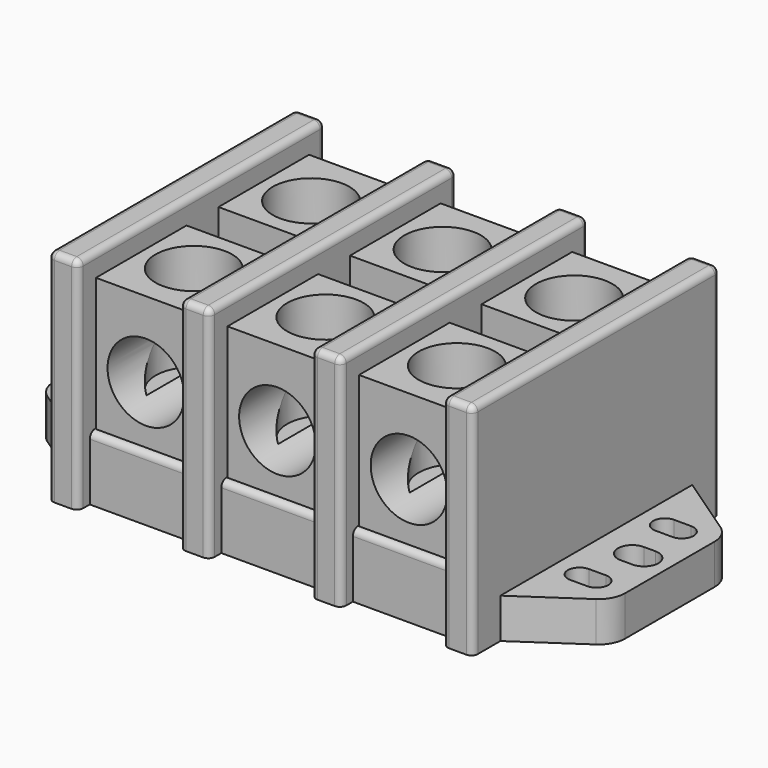
from build123d import *

# Parameters (mm, degrees)
F1_DEPTH  = 52.324
F0_W      = 7.14375
F0_H      = 73.66
F3_DEPTH  = 15.24
F5_DEPTH  = 9.525
F6_R      = 1.524
F6_2_R    = 1.524
F6_3_R    = 1.524
F6_4_R    = 1.524
F6_5_R    = 1.524
F8_DEPTH  = 9.525
F9_W      = 4.064
F9_H      = 5.588
F9_W_2    = 2.794
F9_H_2    = 6.858
F10_DEPTH = 9.525
F11_W     = 2.794
F11_H     = 6.858
F11_W_2   = 4.064
F11_H_2   = 5.588
F12_DEPTH = 9.525
F13_R     = 6.35
F13_2_R   = 6.35
F15_W     = 23.8125
F15_H     = 63.5
F18_DEPTH = 31.75
F16_W     = 23.8125
F16_H     = 63.5
F17_W     = 23.8125
F17_H     = 63.5
F19_R     = 9.128125
F20_DEPTH = 25.4
F21_R     = 9.128125
F22_DEPTH = 25.4
F23_R     = 9.128125
F24_DEPTH = 25.4
F25_W     = 23.8125
F25_H     = 9.525
F26_DEPTH = 18.034
F27_W     = 23.8125
F27_H     = 9.525
F28_DEPTH = 18.034
F29_W     = 23.8125
F29_H     = 9.525
F30_DEPTH = 18.034
F31_R     = 9.144
F32_DEPTH = 26.9875
F33_R     = 9.128125
F34_DEPTH = 26.9875
F35_R     = 9.128125
F36_DEPTH = 26.9875
F37_R     = 9.128125
F38_DEPTH = 26.9875
F39_R     = 9.128125
F40_DEPTH = 26.9875
F41_R     = 9.128125
F42_DEPTH = 26.9875


# Not quite as in the source:
# - a feature names something its author has since deleted; it is built from what else it names


with BuildPart() as f1:
    # F0 (on Top) → F1 (new body)
    with BuildSketch(Plane.XY):
        Polygon((-50.6015625, -36.83), (-43.4578125, -36.83), (-43.4578125, 36.83), (-50.6015625, 36.83), align=None)
    extrude(amount=F1_DEPTH)

    # F4 (on Top) → F5 (join)
    with BuildSketch(Plane.XY):
        Polygon((-50.6015625, -28.575), (-50.6015625, 28.575), (-68.1275625, 16.66875), (-68.1275625, -16.66875), align=None)
    extrude(amount=F5_DEPTH)

    # F6
    f6_edges = [f1.edges().sort_by_distance(p)[0] for p in [
        (-50.601563, 36.83, 26.162),
        (-50.601563, 0, 52.324),
        (-50.601563, -36.83, 26.162),
        (-43.457813, -36.83, 26.162),
        (-43.457813, 0, 52.324),
        (-47.029688, -36.83, 52.324),
        (-47.029687, 36.83, 52.324),
        (-43.457813, 36.83, 26.162),
    ]]
    fillet(f6_edges, radius=F6_R)

    # F9 (on face) → F10 (cut)
    with BuildSketch(Plane.XY.offset(9.525)):
        with Locations((-58.801, 12.7)):
            Rectangle(F9_W, F9_H)
        with BuildLine():
            Line((-56.769, 15.494), (-56.769, 9.906))
            ThreePointArc((-56.769, 9.906), (-53.975, 12.7), (-56.769, 15.494))
        make_face()
        with BuildLine():
            ThreePointArc((-60.833, 15.494), (-63.627, 12.7), (-60.833, 9.906))
            Line((-60.833, 9.906), (-60.833, 15.494))
        make_face()
        with Locations((-60.579, 0)):
            Rectangle(F9_W_2, F9_H_2)
        with BuildLine():
            Line((-59.182, 3.429), (-59.182, -3.429))
            ThreePointArc((-59.182, -3.429), (-55.753, 0), (-59.182, 3.429))
        make_face()
        with BuildLine():
            ThreePointArc((-61.976, 3.429), (-65.405, 0), (-61.976, -3.429))
            Line((-61.976, -3.429), (-61.976, 3.429))
        make_face()
        with Locations((-58.801, -12.7)):
            Rectangle(F9_W, F9_H)
        with BuildLine():
            Line((-56.769, -9.906), (-56.769, -15.494))
            ThreePointArc((-56.769, -15.494), (-53.975, -12.7), (-56.769, -9.906))
        make_face()
        with BuildLine():
            ThreePointArc((-60.833, -9.906), (-63.627, -12.7), (-60.833, -15.494))
            Line((-60.833, -15.494), (-60.833, -9.906))
        make_face()
    extrude(amount=-F10_DEPTH, mode=Mode.SUBTRACT)

    # F13
    f13_edges = [f1.edges().sort_by_distance(p)[0] for p in [
        (-68.127563, 16.66875, 4.7625),
        (-68.127563, -16.66875, 4.7625),
    ]]
    fillet(f13_edges, radius=F13_R)


with BuildPart() as f1b:
    # F0 (on Top) → F1, piece 2 (new body)
    with BuildSketch(Plane.XY):
        Polygon((43.4578125, 36.83), (43.4578125, -36.83), (50.6015625, -36.83), (50.6015625, 36.83), align=None)
    extrude(amount=F1_DEPTH)

    # F6#3
    f6_3_edges = [f1b.edges().sort_by_distance(p)[0] for p in [
        (43.457812, -36.83, 26.162),
        (50.601562, -36.83, 26.162),
        (47.029687, -36.83, 52.324),
        (43.457812, 0, 52.324),
        (50.601562, 0, 52.324),
        (47.029688, 36.83, 52.324),
        (43.457813, 36.83, 26.162),
        (50.601563, 36.83, 26.162),
    ]]
    fillet(f6_3_edges, radius=F6_3_R)

    # F7 (on Top) → F8 (join)
    with BuildSketch(Plane.XY):
        Polygon((68.1275625, 16.66875), (50.6015625, 28.575), (50.6015625, -28.575), (68.1275625, -16.66875), align=None)
    extrude(amount=F8_DEPTH)

    # F11 (on face) → F12 (cut)
    with BuildSketch(Plane.XY.offset(9.525)):
        with Locations((60.579, 0)):
            Rectangle(F11_W, F11_H)
        with BuildLine():
            ThreePointArc((59.182, 3.429), (55.753, 0), (59.182, -3.429))
            Line((59.182, -3.429), (59.182, 3.429))
        make_face()
        with BuildLine():
            Line((61.976, 3.429), (61.976, -3.429))
            ThreePointArc((61.976, -3.429), (65.405, 0), (61.976, 3.429))
        make_face()
        with Locations((58.801, 12.7)):
            Rectangle(F11_W_2, F11_H_2)
        with BuildLine():
            Line((60.833, 15.494), (60.833, 9.906))
            ThreePointArc((60.833, 9.906), (63.627, 12.7), (60.833, 15.494))
        make_face()
        with BuildLine():
            ThreePointArc((56.769, 15.494), (53.975, 12.7), (56.769, 9.906))
            Line((56.769, 9.906), (56.769, 15.494))
        make_face()
        with Locations((58.801, -12.7)):
            Rectangle(F11_W_2, F11_H_2)
        with BuildLine():
            Line((60.833, -9.906), (60.833, -15.494))
            ThreePointArc((60.833, -15.494), (63.627, -12.7), (60.833, -9.906))
        make_face()
        with BuildLine():
            ThreePointArc((56.769, -9.906), (53.975, -12.7), (56.769, -15.494))
            Line((56.769, -15.494), (56.769, -9.906))
        make_face()
    extrude(amount=-F12_DEPTH, mode=Mode.SUBTRACT)

    # F13#2
    f13_2_edges = [f1b.edges().sort_by_distance(p)[0] for p in [
        (68.127562, 16.66875, 4.7625),
        (68.127562, -16.66875, 4.7625),
    ]]
    fillet(f13_2_edges, radius=F13_2_R)


with BuildPart() as f1c:
    # F0 (on Top) → F1, piece 3 (new body)
    with BuildSketch(Plane.XY):
        with Locations((-15.6765625, 0)):
            Rectangle(F0_W, F0_H)
    extrude(amount=F1_DEPTH)

    # F6#4
    f6_4_edges = [f1c.edges().sort_by_distance(p)[0] for p in [
        (-19.248438, 36.83, 26.162),
        (-19.248438, 0, 52.324),
        (-19.248438, -36.83, 26.162),
        (-12.104688, -36.83, 26.162),
        (-15.676563, 36.83, 52.324),
        (-15.676563, -36.83, 52.324),
        (-12.104688, 0, 52.324),
        (-12.104688, 36.83, 26.162),
    ]]
    fillet(f6_4_edges, radius=F6_4_R)


with BuildPart() as f1d:
    # F0 (on Top) → F1, piece 4 (new body)
    with BuildSketch(Plane.XY):
        with Locations((15.6765625, 0)):
            Rectangle(F0_W, F0_H)
    extrude(amount=F1_DEPTH)

    # F6#5
    f6_5_edges = [f1d.edges().sort_by_distance(p)[0] for p in [
        (12.104688, 36.83, 26.162),
        (12.104688, 0, 52.324),
        (12.104688, -36.83, 26.162),
        (19.248438, -36.83, 26.162),
        (19.248438, 0, 52.324),
        (19.248438, 36.83, 26.162),
        (15.676563, -36.83, 52.324),
        (15.676563, 36.83, 52.324),
    ]]
    fillet(f6_5_edges, radius=F6_5_R)


with BuildPart() as f3:
    # F2 (on Top) → F3 (new body)
    with BuildSketch(Plane.XY):
        Polygon((-43.4578125, 33.3375), (-43.4578125, -33.3375), (43.4578125, -33.3375), (43.4578125, 33.3375), align=None)
    extrude(amount=F3_DEPTH)

    # F6#2
    f6_2_edges = [f3.edges().sort_by_distance(p)[0] for p in [
        (0, 33.3375, 15.24),
        (0, -33.3375, 15.24),
    ]]
    fillet(f6_2_edges, radius=F6_2_R)


with BuildPart() as f1_1:
    add(f1.part)

    # F14: union F1b, F1c, F1d, F3
    add(f1b.part)
    add(f1c.part)
    add(f1d.part)
    add(f3.part)


with BuildPart() as f18:
    # F15 (on face) → F18 (new body)
    with BuildSketch(Plane.XY.offset(15.24)):
        with Locations((-31.353125, 0)):
            Rectangle(F15_W, F15_H)
    extrude(amount=F18_DEPTH)

    # F19 (on face) → F20 (cut)
    with BuildSketch(Plane.XY.offset(46.99)):
        with Locations((-31.353125, 17.4625)):
            Circle(F19_R)
        with Locations((-31.353125, -17.4625)):
            Circle(F19_R)
    extrude(amount=-F20_DEPTH, mode=Mode.SUBTRACT)

    # F25 (on face) → F26 (cut)
    with BuildSketch(Plane.XY.offset(46.99)):
        with Locations((-31.353125, 0)):
            Rectangle(F25_W, F25_H)
    extrude(amount=-F26_DEPTH, mode=Mode.SUBTRACT)

    # F31 (on face) → F32 (cut)
    with BuildSketch(Plane.XZ.offset(31.75)):
        with Locations((-31.353125, 28.956)):
            Circle(F31_R)
    extrude(amount=-F32_DEPTH, mode=Mode.SUBTRACT)

    # F41 (on face) → F42 (cut)
    with BuildSketch(Plane(origin=(0, 31.75, 0), x_dir=(-1, 0, 0), z_dir=(0, 1, 0))):
        with Locations((31.353125, 28.956)):
            Circle(F41_R)
    extrude(amount=-F42_DEPTH, mode=Mode.SUBTRACT)


with BuildPart() as f18b:
    # F16 (on face) → F18, piece 2 (new body)
    with BuildSketch(Plane.XY.offset(15.24)):
        Rectangle(F16_W, F16_H)
    extrude(amount=F18_DEPTH)

    # F21 (on face) → F22 (cut)
    with BuildSketch(Plane.XY.offset(46.99)):
        with Locations((0, 17.4625)):
            Circle(F21_R)
        with Locations((0, -17.4625)):
            Circle(F21_R)
    extrude(amount=-F22_DEPTH, mode=Mode.SUBTRACT)

    # F27 (on face) → F28 (cut)
    with BuildSketch(Plane.XY.offset(46.99)):
        Rectangle(F27_W, F27_H)
    extrude(amount=-F28_DEPTH, mode=Mode.SUBTRACT)

    # F33 (on face) → F34 (cut)
    with BuildSketch(Plane.XZ.offset(31.75)):
        with Locations((0, 28.956)):
            Circle(F33_R)
    extrude(amount=-F34_DEPTH, mode=Mode.SUBTRACT)

    # F39 (on face) → F40 (cut)
    with BuildSketch(Plane(origin=(0, 31.75, 0), x_dir=(-1, 0, 0), z_dir=(0, 1, 0))):
        with Locations((0, 28.956)):
            Circle(F39_R)
    extrude(amount=-F40_DEPTH, mode=Mode.SUBTRACT)


with BuildPart() as f18c:
    # F17 (on face) → F18, piece 3 (new body)
    with BuildSketch(Plane.XY.offset(15.24)):
        with Locations((31.353125, 0)):
            Rectangle(F17_W, F17_H)
    extrude(amount=F18_DEPTH)

    # F23 (on face) → F24 (cut)
    with BuildSketch(Plane.XY.offset(46.99)):
        with Locations((31.353125, 17.4625)):
            Circle(F23_R)
        with Locations((31.353125, -17.4625)):
            Circle(F23_R)
    extrude(amount=-F24_DEPTH, mode=Mode.SUBTRACT)

    # F29 (on face) → F30 (cut)
    with BuildSketch(Plane.XY.offset(46.99)):
        with Locations((31.353125, 0)):
            Rectangle(F29_W, F29_H)
    extrude(amount=-F30_DEPTH, mode=Mode.SUBTRACT)

    # F35 (on face) → F36 (cut)
    with BuildSketch(Plane.XZ.offset(31.75)):
        with Locations((31.353125, 28.956)):
            Circle(F35_R)
    extrude(amount=-F36_DEPTH, mode=Mode.SUBTRACT)

    # F37 (on face) → F38 (cut)
    with BuildSketch(Plane(origin=(0, 31.75, 0), x_dir=(-1, 0, 0), z_dir=(0, 1, 0))):
        with Locations((-31.353125, 28.956)):
            Circle(F37_R)
    extrude(amount=-F38_DEPTH, mode=Mode.SUBTRACT)


solid = Compound([f1_1.part, f18.part, f18b.part, f18c.part])
